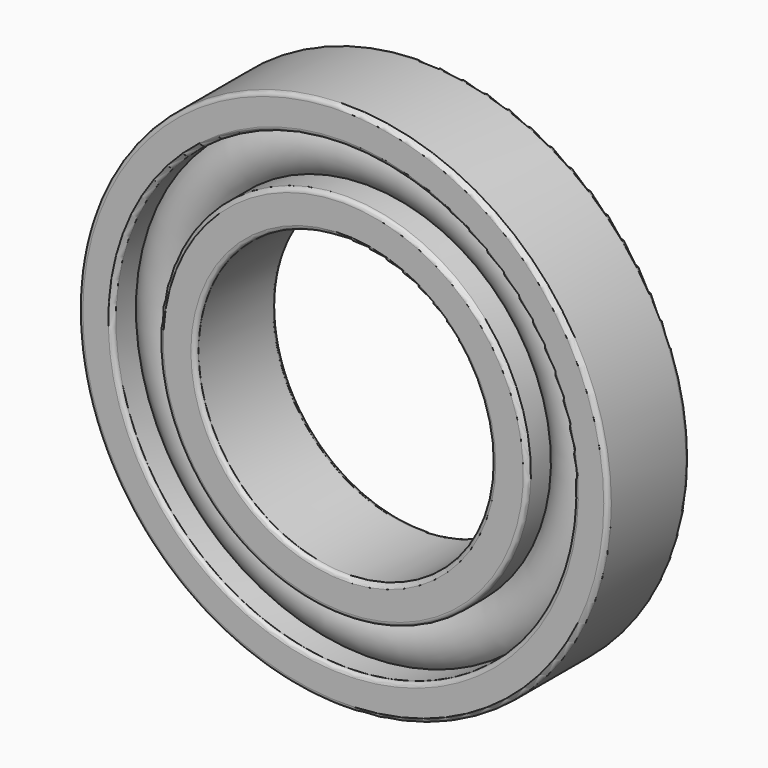
from build123d import *

# Parameters (mm, degrees)
F0_R     = 62.5
F0_R_2   = 35
F1_DEPTH = 12
F4_R     = 1


with BuildPart() as f1:
    # F0 (on Front) → F1 (new body, symmetric)
    with BuildSketch(Plane.XZ):
        Circle(F0_R)
        Circle(F0_R_2, mode=Mode.SUBTRACT)
    extrude(amount=F1_DEPTH, both=True)

    # F2 (on Right) → F3 (revolve, cut)
    with BuildSketch(Plane.YZ):
        with BuildLine():
            Line((-5.0990195136, 54.5), (-22, 54.5))
            Line((-22, 54.5), (-22, 43.5))
            Line((-22, 43.5), (-5.0990195136, 43.5))
            ThreePointArc((-5.0990195136, 43.5), (-7.5, 49), (-5.0990195136, 54.5))
        make_face()
        with BuildLine():
            Line((22, 43.5), (22, 54.5))
            Line((22, 54.5), (5.0990195136, 54.5))
            ThreePointArc((5.0990195136, 54.5), (7.5, 49), (5.0990195136, 43.5))
            Line((5.0990195136, 43.5), (22, 43.5))
        make_face()
    revolve(axis=Axis((0, 16.4881043163, 0), (0, 1, 0)), mode=Mode.SUBTRACT)

    # F4
    f4_edges = [f1.edges().sort_by_distance(p)[0] for p in [
        (-62.5, 12, 0),
        (-62.5, -12, 0),
        (-35, 12, 0),
        (-35, -12, 0),
        (0, -12, -54.5),
        (0, -12, -43.5),
        (0, 12, -54.5),
        (0, 12, -43.5),
    ]]
    fillet(f4_edges, radius=F4_R)


solid = f1.part
